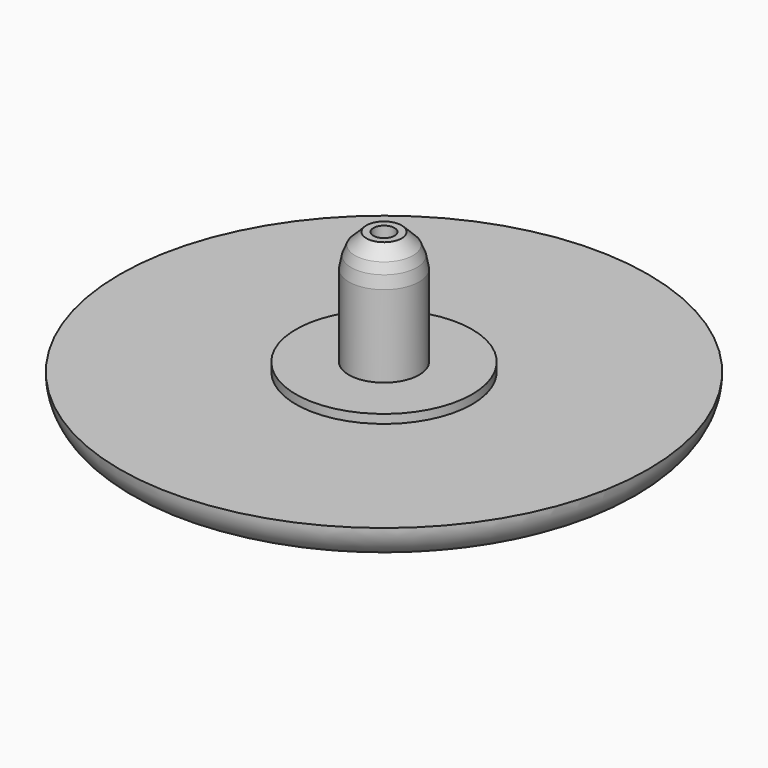
from build123d import *

# Parameters (mm, degrees)
F0_R      = 2
F1_DEPTH  = 7
F2_T      = -1.4
F0_R_2    = 15
F3_DEPTH  = 2
F4_R      = 1.99999
F6_SIZE   = 1
F7_SIZE   = 0.5
F8_SIZE   = 0.35
F9_R      = 5
F9_R_2    = 2
F10_DEPTH = 0.5


# Not quite as in the source:
# - a fillet or chamfer is up to 0.001 mm smaller than in the source, because OpenCascade refuses the exact size


with BuildPart() as f1:
    # F0 (on Top) → F1 (new body)
    with BuildSketch(Plane.XY):
        Circle(F0_R)
    extrude(amount=F1_DEPTH)

    # F2
    f2_openings = [f1.faces().sort_by_distance(p)[0] for p in [
        (0, 0, 7),
    ]]
    offset(amount=F2_T, openings=f2_openings)

    # F0 (on Top) → F3 (join)
    with BuildSketch(Plane.XY):
        Circle(F0_R_2)
        Circle(F0_R, mode=Mode.SUBTRACT)
        Circle(F0_R)
    extrude(amount=-F3_DEPTH)

    # F4 (radius 2 in the source; OpenCascade refuses exactly that, so slightly less here)
    f4_edges = [f1.edges().sort_by_distance(p)[0] for p in [
        (-15, 0, -2),
    ]]
    fillet(f4_edges, radius=F4_R)

    # F6
    f6_edges = [f1.edges().sort_by_distance(p)[0] for p in [
        (-2, 0, 7),
    ]]
    chamfer(f6_edges, length=F6_SIZE)

    # F7
    f7_edges = [f1.edges().sort_by_distance(p)[0] for p in [
        (-2, 0, 6),
    ]]
    chamfer(f7_edges, length=F7_SIZE)

    # F8
    f8_edges = [f1.edges().sort_by_distance(p)[0] for p in [
        (-1.999991, 0, 5.5),
    ]]
    chamfer(f8_edges, length=F8_SIZE)

    # F9 (on face) → F10 (join)
    with BuildSketch(Plane.XY):
        Circle(F9_R)
        Circle(F9_R_2, mode=Mode.SUBTRACT)
    extrude(amount=F10_DEPTH)


solid = f1.part
